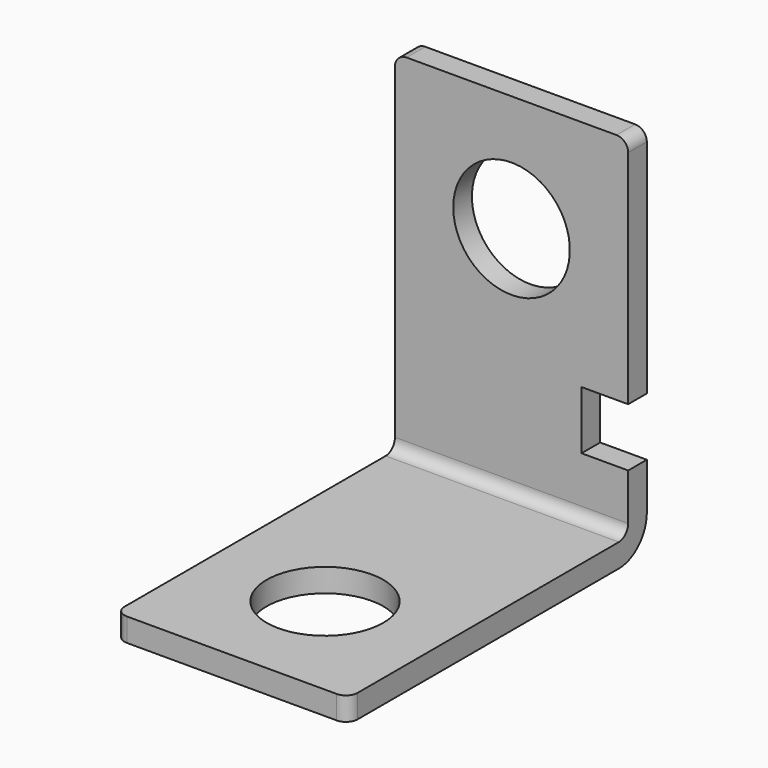
from build123d import *

# Parameters (mm, degrees)
F0_W     = 20
F0_H     = 30
F0_R     = 5
F1_DEPTH = 2
F2_R     = 5
F3_DEPTH = 2
F4_W     = 20
F4_H     = 2
F5_DEPTH = 2
F6_R     = 1
F7_R     = 1
F8_R     = 3


with BuildPart() as f1:
    # F0 (on Top) → F1 (new body)
    with BuildSketch(Plane.XY):
        with Locations((10, 15)):
            Rectangle(F0_W, F0_H)
        with Locations((10, 10)):
            Circle(F0_R, mode=Mode.SUBTRACT)
    extrude(amount=F1_DEPTH)

    # F2 (on face) → F3 (join)
    with BuildSketch(Plane(origin=(0, 30, 0), x_dir=(-1, 0, 0), z_dir=(0, 1, 0))):
        Polygon((-20, 7), (-20, 2), (0, 2), (0, 32), (-20, 32), (-20, 12), (-16, 12), (-16, 7), align=None)
        with Locations((-10, 22)):
            Circle(F2_R, mode=Mode.SUBTRACT)
    extrude(amount=F3_DEPTH)

    # F4 (on face) → F5 (join)
    with BuildSketch(Plane(origin=(0, 30, 0), x_dir=(-1, 0, 0), z_dir=(0, 1, 0))):
        with Locations((-10, 1)):
            Rectangle(F4_W, F4_H)
    extrude(amount=F5_DEPTH)

    # F6
    f6_edges = [f1.edges().sort_by_distance(p)[0] for p in [
        (20, 0, 1),
        (0, 0, 1),
        (20, 31, 32),
        (0, 31, 32),
    ]]
    fillet(f6_edges, radius=F6_R)

    # F7
    f7_edges = [f1.edges().sort_by_distance(p)[0] for p in [
        (10, 30, 2),
    ]]
    fillet(f7_edges, radius=F7_R)

    # F8
    f8_edges = [f1.edges().sort_by_distance(p)[0] for p in [
        (10, 32, 0),
    ]]
    fillet(f8_edges, radius=F8_R)


solid = f1.part
